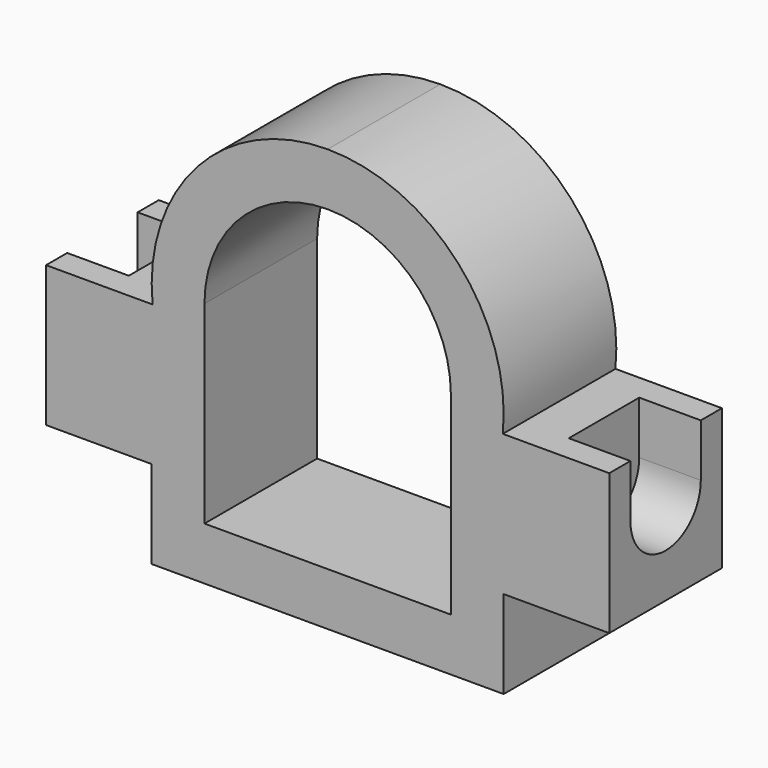
from build123d import *

# Parameters (mm, degrees)
F1_DEPTH = 16
F3_DEPTH = 7


# Not quite as in the source:
# - a pattern or mirror of a feature is missing from the dataset's text; its kind, count and spacing are read off the source's solid


with BuildPart() as f1:
    # F0 (on Front) → F1 (new body)
    with BuildSketch(Plane.XZ):
        with BuildLine():
            Line((-20, 0), (0, 0))
            Line((0, 0), (0, 6))
            Line((0, 6), (-14, 6))
            Line((-14, 6), (-14, 28))
            ThreePointArc((-14, 28), (-9.8994949366, 37.8994949366), (0, 42))
            Line((0, 42), (0, 48))
            ThreePointArc((0, 48), (-14.8323969742, 41.416407865), (-19.8997487421, 26))
            Line((-19.8997487421, 26), (-32, 26))
            Line((-32, 26), (-32, 10))
            Line((-32, 10), (-20, 10))
            Line((-20, 10), (-20, 0))
        make_face()
    extrude(amount=F1_DEPTH)

    # F1_copies: F1 across plane


with BuildPart() as f1_1:
    add(f1.part)
    add(f1.part.mirror(Plane(origin=(0, 0, 0), x_dir=(0, 0, 1), z_dir=(1, 0, 0))))

    # F2 (on face) → F3 (cut)
    with BuildSketch(Plane(origin=(-32, 0, 0), x_dir=(0, -1, 0), z_dir=(-1, 0, 0))):
        with BuildLine():
            Line((13, 26), (3, 26))
            Line((3, 26), (3, 20))
            ThreePointArc((3, 20), (8, 15), (13, 20))
            Line((13, 20), (13, 26))
        make_face()
    f3 = extrude(amount=-F3_DEPTH, mode=Mode.SUBTRACT)

    # F3_copies: F3 across plane
    add(f3.mirror(Plane(origin=(0, 0, 0), x_dir=(0, 0, 1), z_dir=(1, 0, 0))), mode=Mode.SUBTRACT)


solid = f1_1.part
